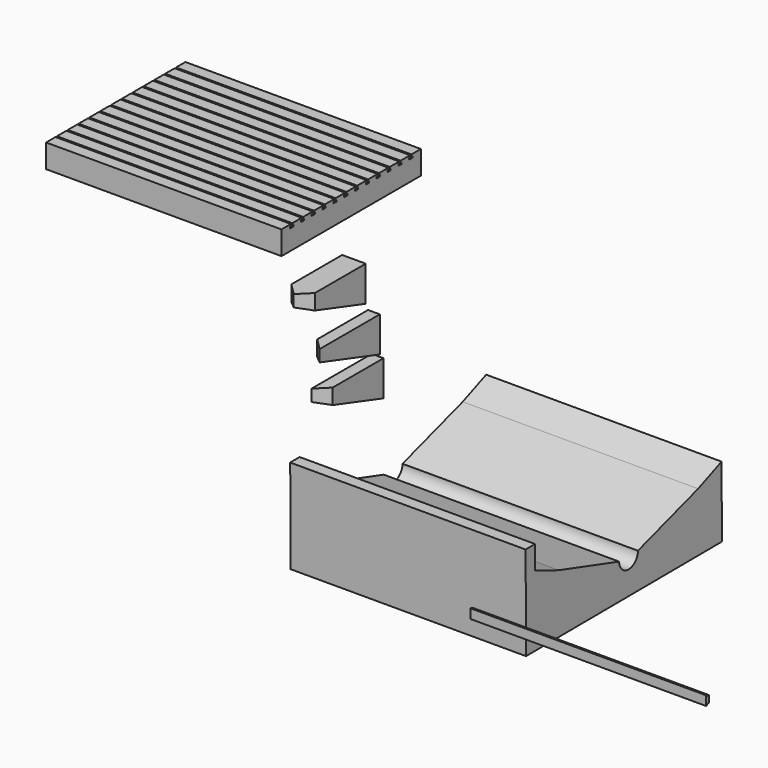
from build123d import *

# Parameters (mm, degrees)
F1_DEPTH  = 2000
F3_DEPTH  = 200
F4_SIZE   = 100
F5_SIZE   = 99.99999
F8_DEPTH  = 100
F9_DEPTH  = 100
F10_SIZE  = 99.99999
F11_SIZE  = 99.99999
F13_DEPTH = 2000
F15_DEPTH = 2000


# Not quite as in the source:
# - a fillet or chamfer is up to 0.001 mm smaller than in the source, because OpenCascade refuses the exact size


with BuildPart() as f1:
    # F0 (on Right) → F1 (new body)
    with BuildSketch(Plane.YZ):
        Polygon((31.3205629587, 15), (-68.6794370413, 15), (-68.6794370413, -185), (1411.3205629587, -185), (1411.3205629587, 15), (1311.3205629587, 15), (1311.3205629587, 0), (1321.3205629587, 0), (1321.3205629587, -15), (1286.3205629587, -15), (1286.3205629587, 0), (1296.3205629587, 0), (1296.3205629587, 15), (1196.3205629587, 15), (1196.3205629587, 0), (1206.3205629587, 0), (1206.3205629587, -15), (1171.3205629587, -15), (1171.3205629587, 0), (1181.3205629587, 0), (1181.3205629587, 15), (1081.3205629587, 15), (1081.3205629587, 0), (1091.3205629587, 0), (1091.3205629587, -15), (1056.3205629587, -15), (1056.3205629587, 0), (1066.3205629587, 0), (1066.3205629587, 15), (966.3205629587, 15), (966.3205629587, 0), (976.3205629587, 0), (976.3205629587, -15), (941.3205629587, -15), (941.3205629587, 0), (951.3205629587, 0), (951.3205629587, 15), (851.3205629587, 15), (851.3205629587, 0), (861.3205629587, 0), (861.3205629587, -15), (826.3205629587, -15), (826.3205629587, 0), (836.3205629587, 0), (836.3205629587, 15), (736.3205629587, 15), (736.3205629587, 0), (746.3205629587, 0), (746.3205629587, -15), (711.3205629587, -15), (711.3205629587, 0), (721.3205629587, 0), (721.3205629587, 15), (621.3205629587, 15), (621.3205629587, 0), (631.3205629587, 0), (631.3205629587, -15), (596.3205629587, -15), (596.3205629587, 0), (606.3205629587, 0), (606.3205629587, 15), (506.3205629587, 15), (506.3205629587, 0), (516.3205629587, 0), (516.3205629587, -15), (481.3205629587, -15), (481.3205629587, 0), (491.3205629587, 0), (491.3205629587, 15), (391.3205629587, 15), (391.3205629587, 0), (401.3205629587, 0), (401.3205629587, -15), (366.3205629587, -15), (366.3205629587, 0), (376.3205629587, 0), (376.3205629587, 15), (276.3205629587, 15), (276.3205629587, 0), (286.3205629587, 0), (286.3205629587, -15), (251.3205629587, -15), (251.3205629587, 0), (261.3205629587, 0), (261.3205629587, 15), (161.3205629587, 15), (161.3205629587, 0), (171.3205629587, 0), (171.3205629587, -15), (136.3205629587, -15), (136.3205629587, 0), (146.3205629587, 0), (146.3205629587, 15), (46.3205629587, 15), (46.3205629587, 0), (56.3205629587, 0), (56.3205629587, -15), (21.3205629587, -15), (21.3205629587, 0), (31.3205629587, 0), align=None)
    extrude(amount=F1_DEPTH)


with BuildPart() as f3:
    # F2 (on face) → F3 (new body)
    with BuildSketch(Plane.YZ.offset(2000)):
        Polygon((575.9602183104, -438.1909608841), (-64.0397816896, -438.1909608841), (-64.0397816896, -538.1909608841), (575.9602183104, -738.1909608841), align=None)
    extrude(amount=F3_DEPTH)

    # F4
    f4_edges = [f3.edges().sort_by_distance(p)[0] for p in [
        (2200, -64.039782, -488.190961),
    ]]
    chamfer(f4_edges, length=F4_SIZE)

    # F5 (size 100 in the source; OpenCascade refuses exactly that, so slightly less here)
    f5_edges = [f3.edges().sort_by_distance(p)[0] for p in [
        (2000, -64.039782, -488.190961),
    ]]
    chamfer(f5_edges, length=F5_SIZE)


with BuildPart() as f8:
    # F6 (on face) → F8 (new body)
    with BuildSketch(Plane.YZ.offset(2200)):
        Polygon((600.5844579637, -1094.5291638374), (600.5844579637, -794.5291638374), (-39.4155420363, -794.5291638374), (-39.4155420363, -894.5291638374), align=None)
    extrude(amount=F8_DEPTH)

    # F10 (size 100 in the source; OpenCascade refuses exactly that, so slightly less here)
    f10_edges = [f8.edges().sort_by_distance(p)[0] for p in [
        (2200, -39.415542, -844.529164),
    ]]
    chamfer(f10_edges, length=F10_SIZE)


with BuildPart() as f9:
    # F7 (on face) → F9 (new body)
    with BuildSketch(Plane.YZ.offset(2200)):
        Polygon((640, -1438.8029098511), (640, -1138.8029098511), (0, -1138.8029098511), (0, -1238.8029098511), align=None)
    extrude(amount=F9_DEPTH)

    # F11 (size 100 in the source; OpenCascade refuses exactly that, so slightly less here)
    f11_edges = [f9.edges().sort_by_distance(p)[0] for p in [
        (2300, 0, -1188.80291),
    ]]
    chamfer(f11_edges, length=F11_SIZE)


with BuildPart() as f13:
    # F12 (on face) → F13 (new body)
    with BuildSketch(Plane.YZ.offset(2300)):
        with BuildLine():
            ThreePointArc((841.7896378459, -2010.1940166026), (741.7914475541, -2109.592403471), (641.7932572623, -2010.1940166026))
            Line((641.7932572623, -2010.1940166026), (0.6016131315, -1814.0479600607))
            Line((0.6016131315, -1814.0479600607), (-249.9954757296, -1715.5538025978))
            Line((-249.9954757296, -1715.5538025978), (-251.1987019926, -1515.5574220141))
            Line((-251.1987019926, -1515.5574220141), (-351.1968922845, -1516.1590351456))
            Line((-351.1968922845, -1516.1590351456), (-346.3839872322, -2316.1445574802))
            Line((-346.3839872322, -2316.1445574802), (-246.3857969404, -2315.5429443487))
            Line((-246.3857969404, -2315.5429443487), (1733.5783708378, -2304.8342306074))
            Line((1733.5783708378, -2304.8342306074), (1729.9686920486, -1704.8450888564))
            Line((1729.9686920486, -1704.8450888564), (1480.5748294505, -1806.3473119771))
            Line((1480.5748294505, -1806.3473119771), (841.7896378459, -2010.1940166026))
        make_face()
    extrude(amount=F13_DEPTH)


with BuildPart() as f15:
    # F14 (on face) → F15 (new body)
    with BuildSketch(Plane.YZ.offset(4300)):
        Polygon((-925.4759454727, -1718.6972332001), (-935.4759454727, -1718.6972332001), (-935.4759454727, -1798.6972332001), (-925.4759454727, -1798.6972332001), (-925.4759454727, -1788.6972332001), (-905.4759454727, -1788.6972332001), (-905.4759454727, -1728.6972332001), (-925.4759454727, -1728.6972332001), align=None)
    extrude(amount=F15_DEPTH)


solid = Compound([f1.part, f3.part, f8.part, f9.part, f13.part, f15.part])
